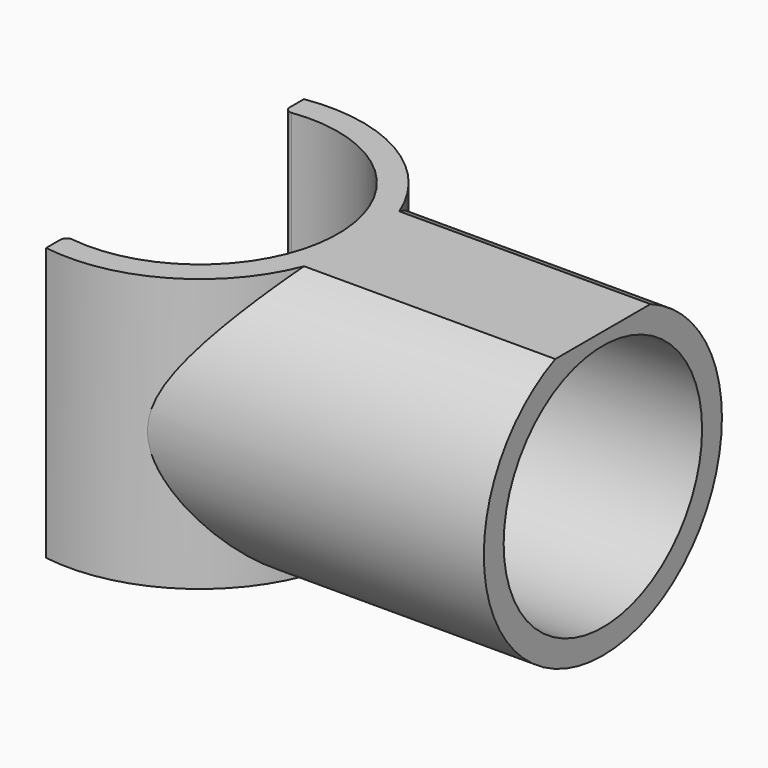
from build123d import *

# Parameters (mm, degrees)
F1_DEPTH      = 11
F1_DEPTH_BACK = 11
F2_R          = 10
F3_DEPTH      = 25
F6_END_RADIUS = 13.15
F5_R          = 12
F5_R_2        = 10
F6_REACH      = 68.442125597
F7_T4_ANGLE   = 86.3533795546
F7_S5_R       = 12
F7_T6_DEPTH   = 12
F8_W          = 15.702219009
F8_H          = 5.1735627732
F9_DEPTH      = 32.5010001


# Not quite as in the source:
# - a fillet or chamfer that OpenCascade refuses, or shapes differently, is made with other operations: its cross-section is extruded or revolved along the edge and cut away or added


with BuildPart() as f1:
    # F0 (on Top) → F1 (new body, two sides)
    with BuildSketch(Plane.XY) as f1_sk:
        with BuildLine():
            ThreePointArc((-1.4356223176, 11.0571917122), (11.15, 0), (-1.4356223176, -11.0571917122))
            ThreePointArc((-1.4356223176, -11.0571917122), (-1.8300084535, -11.1774045329), (-2, -11.5530299056))
            Line((-2, -11.5530299056), (-2, -12.997018889))
            ThreePointArc((-2, -12.997018889), (13.15, 0), (-2, 12.997018889))
            Line((-2, 12.997018889), (-2, 11.5530299056))
            ThreePointArc((-2, 11.5530299056), (-1.8300084535, 11.1774045329), (-1.4356223176, 11.0571917122))
        make_face()
    extrude(amount=F1_DEPTH)
    extrude(f1_sk.sketch, amount=-F1_DEPTH_BACK)

    # F2 (on Right) → F3 (cut)
    with BuildSketch(Plane.YZ):
        Circle(F2_R)
    extrude(amount=F3_DEPTH, mode=Mode.SUBTRACT)

    f6_end = (Plane(origin=(0, 0, 0), x_dir=(-1, 0, 0), z_dir=(0, 0, -1)) * Cylinder(F6_END_RADIUS, 211.856580101, mode=Mode.PRIVATE)).faces().sort_by_distance((13.15, 0, 10.6251383555))[0]
    # F5 (on offset) → F6 (join, up to the whole of a round face its end follows)
    with BuildSketch(Plane.YZ.offset(32.5)):
        Circle(F5_R)
        Circle(F5_R_2, mode=Mode.SUBTRACT)
    f6_long = extrude(amount=-F6_REACH, mode=Mode.PRIVATE)
    add(split(f6_long, bisect_by=f6_end, keep=Keep.ALL, mode=Mode.PRIVATE).solids().sort_by_distance((32.5, -11.660588745, 0))[0])

    # F7: fillet of radius 2 on 1 edges, made by hand


with BuildPart() as f7_tool2:
    # F7_s3 → F7_t4 (revolve)
    with BuildSketch(Plane(origin=(0, 0, 0), x_dir=(0, 0, 1), z_dir=(-0.6842504755, -0.7292470684, 0))):
        with BuildLine():
            ThreePointArc((-11, -11.15), (-11.5857864376, -12.5642135624), (-13, -13.15))
            Line((-13, -13.15), (-11, -13.15))
            Line((-11, -13.15), (-11, -11.15))
        make_face()
    revolve(axis=Axis((0, 0, -11), (0, 0, 1)), revolution_arc=F7_T4_ANGLE)

    # F7_s5 → F7_t6 (intersect, symmetric)
    with BuildSketch(Plane.YZ.offset(10.7)):
        Circle(F7_S5_R)
    extrude(amount=F7_T6_DEPTH, both=True, mode=Mode.INTERSECT)


with BuildPart() as f1_1:
    add(f1.part)

    # F7_t1: union F7_tool2
    add(f7_tool2.part)

    # F8 (on Right) → F9 (cut, through all)
    with BuildSketch(Plane.YZ):
        with Locations((0.481082825, 13.5867813866)):
            Rectangle(F8_W, F8_H)
    extrude(amount=F9_DEPTH, mode=Mode.SUBTRACT)


solid = f1_1.part
